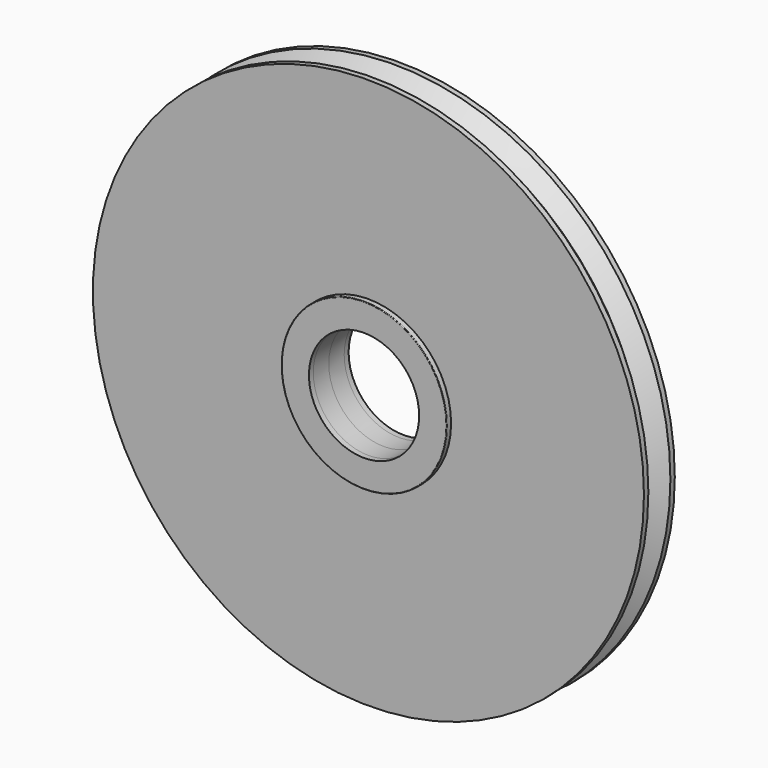
from build123d import *
from build123d import SkipClean  # not in build123d's __all__

# Parameters (mm, degrees)
F0_R     = 50
F1_DEPTH = 3.5
F2_SIZE  = 2.5
F3_R     = 10.0003114876
F4_DEPTH = 3.5
F6_R     = 15
F6_R_2   = 10.0003114876
F7_DEPTH = 1
F8_R     = 15.0083101608
F8_R_2   = 10.0003114876
F9_DEPTH = 1
F10_R    = 0.1


with BuildPart() as f1:
    # F0 (on Front) → F1 (new body)
    with BuildSketch(Plane.XZ):
        Circle(F0_R)
    extrude(amount=F1_DEPTH)

    # F2
    f2_edges = [f1.edges().sort_by_distance(p)[0] for p in [
        (-50, -3.5, 0),
    ]]
    chamfer(f2_edges, length=F2_SIZE)

    # F3 (on face) → F4 (cut)
    with BuildSketch(Plane(origin=(0, 0, 0), x_dir=(-1, 0, 0), z_dir=(0, 1, 0))):
        Circle(F3_R)
    extrude(amount=-F4_DEPTH, mode=Mode.SUBTRACT)

    # F5: F1 across face


with BuildPart() as f1_1:
    add(f1.part, clean=False)
    add(f1.part.mirror(Plane.XZ.offset(3.5)), clean=False)

    # F6 (on face) → F7 (join)
    with BuildSketch(Plane.XZ.offset(7)):
        Circle(F6_R)
        Circle(F6_R_2, mode=Mode.SUBTRACT)
    with SkipClean():  # cleaning this boolean's faces spoils the solid; the shape is the same uncleaned
        extrude(amount=F7_DEPTH)

    # F8 (on face) → F9 (join)
    with BuildSketch(Plane(origin=(0, 0, 0), x_dir=(-1, 0, 0), z_dir=(0, 1, 0))):
        Circle(F8_R)
        Circle(F8_R_2, mode=Mode.SUBTRACT)
    extrude(amount=F9_DEPTH)

    # F10
    f10_edges = [f1_1.edges().sort_by_distance(p)[0] for p in [
        (-15, -8, 0),
        (15.00831, 1, 0),
    ]]
    fillet(f10_edges, radius=F10_R)


solid = f1_1.part
